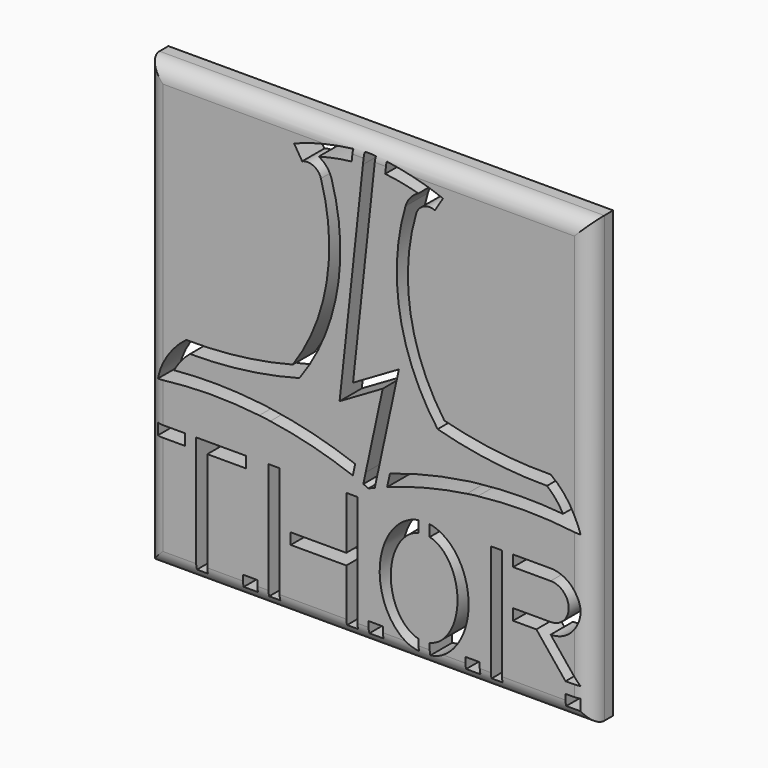
from build123d import *

# Parameters (mm, degrees)
F0_W        = 101.6
F0_H        = 101.6
F1_DEPTH    = 6.35
F2_W        = 6.35
F2_H        = 2.54
F2_W_2      = 3.2650283397
F2_W_3      = 3.2766
F3_DEPTH    = 25.4
F5_DEPTH    = 25.4
F7_DEPTH    = 6.35
F8_T1_DEPTH = 120.65
F8_T3_DEPTH = 120.65


# Not quite as in the source:
# - a fillet or chamfer that OpenCascade refuses, or shapes differently, is made with other operations: its cross-section is extruded or revolved along the edge and cut away or added


with BuildPart() as f1:
    # F0 (on Front) → F1 (new body)
    with BuildSketch(Plane.XZ):
        Rectangle(F0_W, F0_H)
    extrude(amount=F1_DEPTH)

    # F2 (on face) → F3 (cut)
    with BuildSketch(Plane.XZ.offset(6.35)):
        with Locations((-45.085, -22.86)):
            Rectangle(F2_W, F2_H)
        Polygon((-27.94, -24.13), (-27.94, -21.59), (-39.37, -21.59), (-39.37, -24.13), (-39.37, -48.26), (-36.83, -48.26), (-36.83, -24.13), align=None)
        Polygon((-20.32, -21.59), (-22.86, -21.59), (-22.86, -48.26), (-20.32, -48.26), (-20.32, -36.195), (-20.32, -33.655), align=None)
        Polygon((-2.54, -21.59), (-5.08, -21.59), (-5.08, -33.655), (-17.78, -33.655), (-17.78, -36.195), (-5.08, -36.195), (-5.08, -48.26), (-2.54, -48.26), align=None)
        with BuildLine():
            Line((11.43, -24.2809864569), (11.43, -21.6945898501))
            add(Edge.make_bspline(
                [(11.43, -21.6945898501), (2.54, -23.1646354223), (2.54, -34.925), (2.54, -46.6853645777), (11.43, -48.1554101499)],
                knots=[0.1253278312, 0.1253278312, 0.1253278312, 1.5707963268, 1.5707963268, 3.0162648224, 3.0162648224, 3.0162648224], degree=2, weights=[1, 0.75, 1, 0.75, 1]))
            Line((11.43, -48.1554101499), (11.43, -45.5690135431))
            add(Edge.make_bspline(
                [(11.43, -24.2809864569), (5.08, -25.8015598202), (5.08, -34.925), (5.08, -44.0484401798), (11.43, -45.5690135431)],
                knots=[0.1674480792, 0.1674480792, 0.1674480792, 1.5707963268, 1.5707963268, 2.9741445744, 2.9741445744, 2.9741445744], degree=2, weights=[1, 0.7637626158, 1, 0.7637626158, 1]))
        make_face()
        Polygon((30.48, -21.59), (27.94, -21.59), (27.94, -48.26), (30.48, -48.26), (30.48, -34.925), (30.48, -32.385), (30.48, -24.13), align=None)
        with BuildLine():
            Line((48.26, -43.18), (41.5925, -34.925))
            ThreePointArc((41.5925, -34.925), (48.26, -28.2575), (41.5925, -21.59))
            Line((41.5925, -21.59), (33.02, -21.59))
            Line((33.02, -21.59), (33.02, -24.13))
            Line((33.02, -24.13), (41.5925, -24.13))
            ThreePointArc((41.5925, -24.13), (45.72, -28.2575), (41.5925, -32.385))
            Line((41.5925, -32.385), (33.02, -32.385))
            Line((33.02, -32.385), (33.02, -34.925))
            Line((33.02, -34.925), (38.3274716603, -34.925))
            Line((38.3274716603, -34.925), (44.9949716603, -43.18))
            Line((44.9949716603, -43.18), (48.26, -43.18))
        make_face()
        with BuildLine():
            ThreePointArc((24.974716025, -12.4850096138), (36.6248087332, -11.8643810123), (48.26, -12.7200469264))
            ThreePointArc((48.26, -12.7200469264), (45.8270939674, -7.1374713188), (41.6333100019, -2.7220032545))
            ThreePointArc((41.6333100019, -2.7220032545), (29.3742602236, -2.0674257454), (17.313242312, 0.2226878143))
            ThreePointArc((17.313242312, 0.2226878143), (9.5821881501, 19.2515838935), (10.8807589859, 39.7499203682))
            ThreePointArc((10.8807589859, 39.7499203682), (12.5646356449, 41.7283092602), (15.1613568887, 41.8089441955))
            Line((15.1613568887, 41.8089441955), (17.0036368072, 44.7891056538))
            ThreePointArc((17.0036368072, 44.7891056538), (9.2713106692, 47.1161749586), (1.27, 48.2039003973))
            ThreePointArc((1.27, 48.2039003973), (0, 48.2749433866), (-1.27, 48.2039003973))
            ThreePointArc((-1.27, 48.2039003973), (-9.2713106692, 47.1161749586), (-17.0036368072, 44.7891056538))
            Line((-17.0036368072, 44.7891056538), (-15.1613568887, 41.8089441955))
            ThreePointArc((-15.1613568887, 41.8089441955), (-12.5646356449, 41.7283092602), (-10.8807589859, 39.7499203682))
            ThreePointArc((-10.8807589859, 39.7499203682), (-9.5821881501, 19.2515838935), (-17.313242312, 0.2226878143))
            ThreePointArc((-17.313242312, 0.2226878143), (-29.3742602236, -2.0674257454), (-41.6333100019, -2.7220032545))
            ThreePointArc((-41.6333100019, -2.7220032545), (-45.8270939674, -7.1374713188), (-48.26, -12.7200469264))
            ThreePointArc((-48.26, -12.7200469264), (-36.6248087332, -11.8643810123), (-24.974716025, -12.4850096138))
            ThreePointArc((-24.974716025, -12.4850096138), (-23.7004956404, -12.6194303374), (-22.434716025, -12.8181977514))
            ThreePointArc((-22.434716025, -12.8181977514), (-11.0198286809, -15.2229860571), (0, -19.05))
            ThreePointArc((0, -19.05), (11.0198286809, -15.2229860571), (22.434716025, -12.8181977514))
            ThreePointArc((22.434716025, -12.8181977514), (23.7004956404, -12.6194303374), (24.974716025, -12.4850096138))
        make_face()
        with BuildLine():
            ThreePointArc((40.7690218184, -5.2698750692), (42.8084658363, -7.3195469158), (44.4172002099, -9.7221414084))
            ThreePointArc((44.4172002099, -9.7221414084), (34.69065921, -9.3250013889), (24.974716025, -9.9281332518))
            ThreePointArc((24.974716025, -9.9281332518), (23.7015296227, -10.0652142294), (22.434716025, -10.2522386079))
            ThreePointArc((22.434716025, -10.2522386079), (11.0311805947, -12.5864744285), (0, -16.3016233979))
            ThreePointArc((0, -16.3016233979), (-11.0311805947, -12.5864744285), (-22.434716025, -10.2522386079))
            ThreePointArc((-22.434716025, -10.2522386079), (-23.7015296227, -10.0652142294), (-24.974716025, -9.9281332518))
            ThreePointArc((-24.974716025, -9.9281332518), (-34.69065921, -9.3250013889), (-44.4172002099, -9.7221414084))
            ThreePointArc((-44.4172002099, -9.7221414084), (-42.8084658363, -7.3195469158), (-40.7690218184, -5.2698750692))
            ThreePointArc((-40.7690218184, -5.2698750692), (-28.1631581391, -4.4748709965), (-15.7776089495, -1.997371884))
            ThreePointArc((-15.7776089495, -1.997371884), (-7.1527941696, 18.3806886827), (-8.4452652822, 40.4710101125))
            ThreePointArc((-8.4452652822, 40.4710101125), (-9.5514326446, 42.5310335514), (-11.3868656194, 43.9796496486))
            ThreePointArc((-11.3868656194, 43.9796496486), (-6.3726185079, 45.0857261304), (-1.27, 45.6596282487))
            ThreePointArc((-1.27, 45.6596282487), (0, 45.703530978), (1.27, 45.6596282487))
            ThreePointArc((1.27, 45.6596282487), (6.3726185079, 45.0857261304), (11.3868656194, 43.9796496486))
            ThreePointArc((11.3868656194, 43.9796496486), (9.5514326446, 42.5310335514), (8.4452652822, 40.4710101125))
            ThreePointArc((8.4452652822, 40.4710101125), (7.1527941696, 18.3806886827), (15.7776089495, -1.997371884))
            ThreePointArc((15.7776089495, -1.997371884), (28.1631581391, -4.4748709965), (40.7690218184, -5.2698750692))
        make_face(mode=Mode.SUBTRACT)
        with BuildLine():
            Line((13.97, -21.6945898501), (13.97, -24.2809864569))
            add(Edge.make_bspline(
                [(13.97, -45.5690135431), (20.32, -44.0484401798), (20.32, -34.925), (20.32, -25.8015598202), (13.97, -24.2809864569)],
                knots=[3.3090407328, 3.3090407328, 3.3090407328, 4.7123889804, 4.7123889804, 6.115737228, 6.115737228, 6.115737228], degree=2, weights=[1, 0.7637626158, 1, 0.7637626158, 1]))
            Line((13.97, -45.5690135431), (13.97, -48.1554101499))
            add(Edge.make_bspline(
                [(13.97, -48.1554101499), (22.86, -46.6853645777), (22.86, -34.925), (22.86, -23.1646354223), (13.97, -21.6945898501)],
                knots=[3.2669204848, 3.2669204848, 3.2669204848, 4.7123889804, 4.7123889804, 6.157857476, 6.157857476, 6.157857476], degree=2, weights=[1, 0.75, 1, 0.75, 1]))
        make_face()
        with Locations((46.6274858301, -46.99)):
            Rectangle(F2_W_2, F2_H)
        with Locations((23.7617, -46.99)):
            Rectangle(F2_W_3, F2_H)
        with Locations((-27.0383, -46.99)):
            Rectangle(F2_W_3, F2_H)
        with Locations((1.6566223747, -46.99)):
            Rectangle(F2_W_3, F2_H)
    extrude(amount=-F3_DEPTH, mode=Mode.SUBTRACT)

    # F4 (on face) → F5 (cut)
    with BuildSketch(Plane.XZ.offset(6.35)):
        Polygon((6.9247632937, 7.1449134929), (-3.5475781909, 1.0572041649), (1.2626479568, 45.5670753547), (1.3561621326, 46.4323785214), (-1.2626479568, 45.8399866013), (-6.6124218091, -3.662414689), (3.2352367063, 2.0621582436), (-0.7587190834, -16.5345300494), (1.7103416933, -17.1345172863), align=None)
    extrude(amount=-F5_DEPTH, mode=Mode.SUBTRACT)

    # F6 (on face) → F7 (join)
    with BuildSketch(Plane.XZ.offset(6.35)):
        Polygon((-3.972564338, 44.4045720898), (-1.2822182184, 45.6588995184), (-0.9534420353, 48.7011235446), (-3.478737949, 48.9740347912), align=None)
        Polygon((1.6887252067, 49.5096433188), (1.272633295, 45.6594714508), (3.7333616999, 44.7891056538), (4.2140211204, 49.2367320722), align=None)
        Polygon((-1.4639124956, -19.8180571495), (-0.3777049332, -14.7604489729), (-2.6673084195, -13.3248712922), (-3.8673687775, -18.9126017493), align=None)
        Polygon((5.0970298852, -13.4618405507), (2.2202133293, -14.7604489729), (1.0234040391, -20.3330417827), (3.6213223017, -20.3330417827), align=None)
    extrude(amount=-F7_DEPTH)

    # F8: fillet of radius 3.81 on 4 edges, made by hand

    # F8_s2 → F8_t1 (cut)
    with BuildSketch(Plane.XY.offset(-60.325)):
        with BuildLine():
            ThreePointArc((50.8, -2.54), (49.6840768363, -5.2340768363), (46.99, -6.35))
            Line((46.99, -6.35), (50.8, -6.35))
            Line((50.8, -6.35), (50.8, -2.54))
        make_face()
        with BuildLine():
            ThreePointArc((-46.99, -6.35), (-49.6840768363, -5.2340768363), (-50.8, -2.54))
            Line((-50.8, -2.54), (-50.8, -6.35))
            Line((-50.8, -6.35), (-46.99, -6.35))
        make_face()
    extrude(amount=F8_T1_DEPTH, mode=Mode.SUBTRACT)

    # F8_s4 → F8_t3 (cut)
    with BuildSketch(Plane.YZ.offset(-60.325)):
        with BuildLine():
            ThreePointArc((-6.35, -46.99), (-5.2340768363, -49.6840768363), (-2.54, -50.8))
            Line((-2.54, -50.8), (-6.35, -50.8))
            Line((-6.35, -50.8), (-6.35, -46.99))
        make_face()
        with BuildLine():
            ThreePointArc((-6.35, 46.99), (-5.2340768363, 49.6840768363), (-2.54, 50.8))
            Line((-2.54, 50.8), (-6.35, 50.8))
            Line((-6.35, 50.8), (-6.35, 46.99))
        make_face()
    extrude(amount=F8_T3_DEPTH, mode=Mode.SUBTRACT)


solid = f1.part
